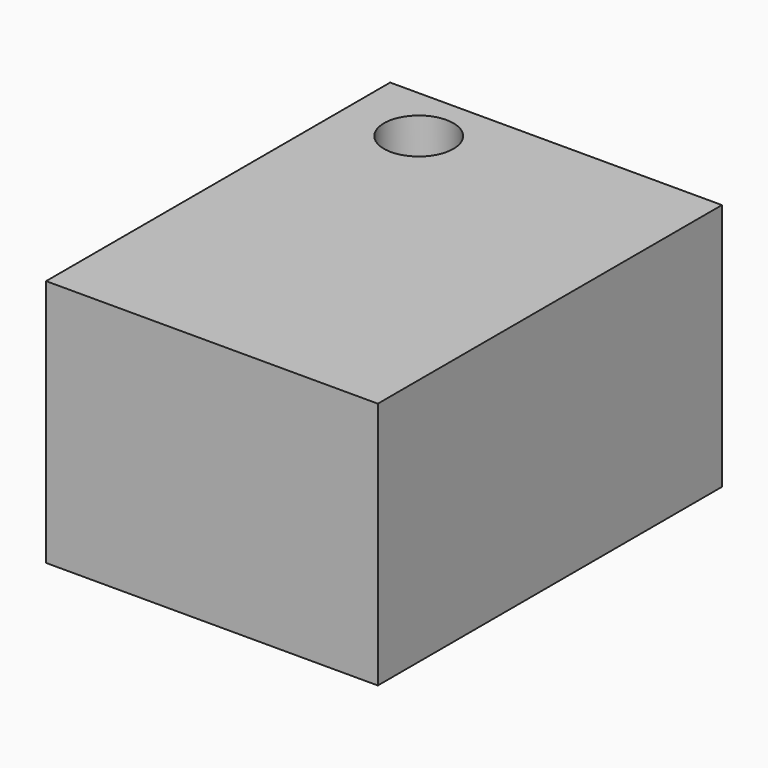
from build123d import *

# Parameters (mm, degrees)
F0_W     = 67.9279565811
F0_H     = 88.0647003651
F1_DEPTH = 25.4
F2_R     = 7.1128535292
F3_DEPTH = 50.801


# Not quite as in the source:
# - a feature of the source that left no trace in its solid (it failed there, or was rolled back) is left out


with BuildPart() as f1:
    # F0 (on Top) → F1 (new body, symmetric)
    with BuildSketch(Plane.XY):
        Rectangle(F0_W, F0_H)
    extrude(amount=F1_DEPTH, both=True)

    # F2 (on face) → F3 (cut, through all)
    with BuildSketch(Plane.XY.offset(25.4)):
        with Locations((-18.8261009753, 32.4227437377)):
            Circle(F2_R)
    extrude(amount=-F3_DEPTH, mode=Mode.SUBTRACT)


solid = f1.part
